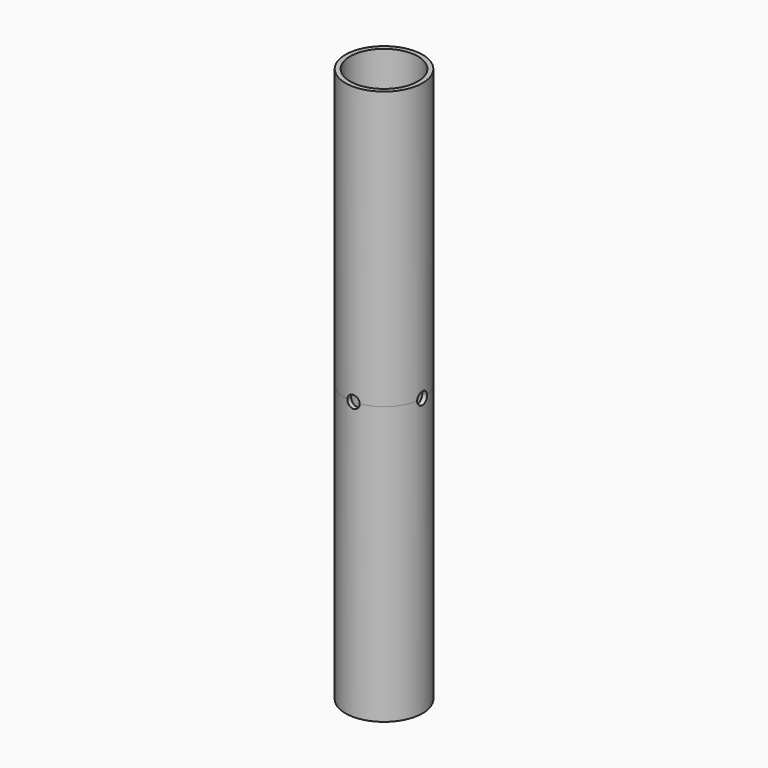
from build123d import *

# Parameters (mm, degrees)
F0_R     = 25
F0_R_2   = 22
F1_DEPTH = 90
F2_DEPTH = 90
F3_R     = 4
F4_DEPTH = 25
F5_DEPTH = 25
F6_R     = 4
F7_DEPTH = 25
F8_DEPTH = 25


# Not quite as in the source:
# - a feature names something its author has since deleted; it is built from what else it names


with BuildPart() as f1:
    # F0 (on Top) → F1 (new body)
    with BuildSketch(Plane.XY):
        Circle(F0_R)
        Circle(F0_R_2, mode=Mode.SUBTRACT)
    extrude(amount=F1_DEPTH)

    # F2 (add): a face of the model
    f2_faces = [f1.faces().sort_by_distance(p)[0] for p in [
        (-24.2928932188, 0, 90),
    ]]
    extrude(f2_faces, amount=F2_DEPTH)

    # F3 (on Right) → F4 (cut)
    with BuildSketch(Plane.YZ):
        Circle(F3_R)
    extrude(amount=F4_DEPTH, mode=Mode.SUBTRACT)

    # F3 (on Right) → F5 (cut)
    with BuildSketch(Plane.YZ):
        Circle(F3_R)
    extrude(amount=-F5_DEPTH, mode=Mode.SUBTRACT)

    # F6 (on Front) → F7 (cut)
    with BuildSketch(Plane.XZ):
        Circle(F6_R)
    extrude(amount=F7_DEPTH, mode=Mode.SUBTRACT)

    # F6 (on Front) → F8 (cut)
    with BuildSketch(Plane.XZ):
        Circle(F6_R)
    extrude(amount=-F8_DEPTH, mode=Mode.SUBTRACT)

    # F9: F1 across plane


with BuildPart() as f1_1:
    add(f1.part)
    add(f1.part.mirror(Plane.XY))


solid = f1_1.part
